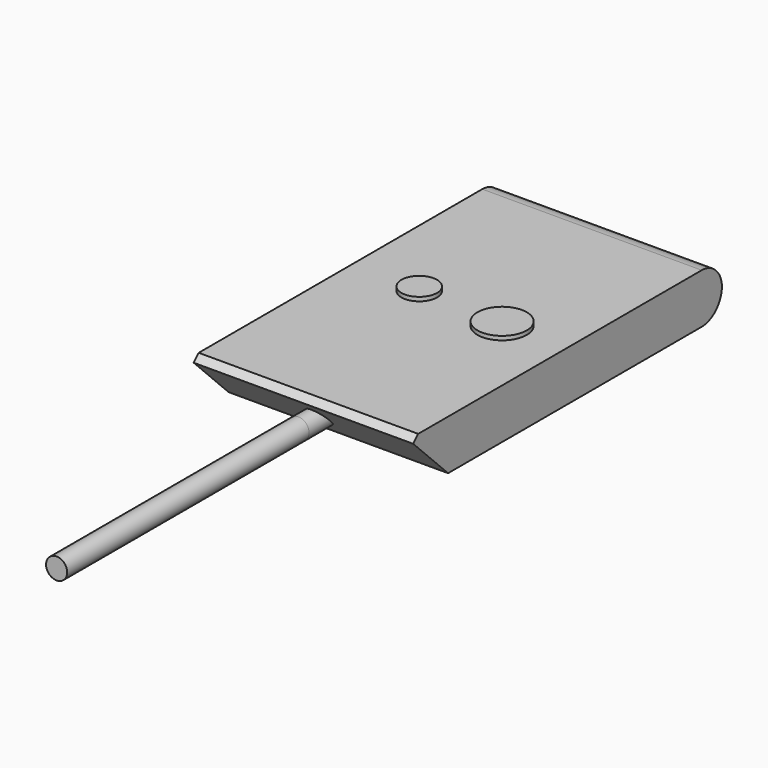
from build123d import *

# Parameters (mm, degrees)
F0_W         = 22.3715566099
F0_H         = 39.9701632559
F1_DEPTH     = 5.08
F2_R         = 5.7912
F3_DEPTH     = 0.762
F4_R         = 1.0769741324
F5_DEPTH     = 50.8
F6_R         = 1.8127400762
F6_R_2       = 2.5138312633
F7_DEPTH     = 0.4064
F8_SIZE      = 1.27
F9_T4_DEPTH  = 48.4998557676
F9_S5_R      = 1.0769741324
F9_T6_DEPTH  = 26
F10_SIZE     = 1.524
F11_T1_DEPTH = 27.632068852


# Not quite as in the source:
# - a fillet or chamfer that OpenCascade refuses, or shapes differently, is made with other operations: its cross-section is extruded or revolved along the edge and cut away or added


with BuildPart() as f1:
    # F0 (on Top) → F1 (new body)
    with BuildSketch(Plane.XY):
        Rectangle(F0_W, F0_H)
    extrude(amount=F1_DEPTH)

    # F2 (on Top) → F3 (cut)
    with BuildSketch(Plane.XY):
        Circle(F2_R)
    extrude(amount=F3_DEPTH, mode=Mode.SUBTRACT)

    # F4 (on Front) → F5 (join)
    with BuildSketch(Plane.XZ):
        with Locations((0, 2.4075380061)):
            Circle(F4_R)
    extrude(amount=F5_DEPTH)

    # F6 (on face) → F7 (join)
    with BuildSketch(Plane.XY.offset(5.08)):
        with Locations((-4.1463463567, 0.584599562)):
            Circle(F6_R)
        with Locations((4.7694612294, 0)):
            Circle(F6_R_2)
    extrude(amount=F7_DEPTH)

    # F8
    f8_edges = [f1.edges().sort_by_distance(p)[0] for p in [
        (0, -19.985082, 5.08),
    ]]
    chamfer(f8_edges, length=F8_SIZE)

    # F9: chamfer of 5.08 on 1 edges, made by hand


with BuildPart() as f9_tool2:
    # F9_s3 → F9_t4 (new body)
    with BuildSketch(Plane.YZ.offset(-24.2499278838)):
        Polygon((-19.985081628, 5.08), (-14.905081628, 0), (-19.985081628, 0), align=None)
    extrude(amount=F9_T4_DEPTH)

    # F9_s5 → F9_t6 (cut, symmetric)
    with BuildSketch(Plane.XZ.offset(17.4)):
        with Locations((0, 2.4075380061)):
            Circle(F9_S5_R)
    extrude(amount=F9_T6_DEPTH, both=True, mode=Mode.SUBTRACT)


with BuildPart() as f1_1:
    add(f1.part)

    # F9_t1: cut F9_tool2
    add(f9_tool2.part, mode=Mode.SUBTRACT)

    # F10
    f10_edges = [f1_1.edges().sort_by_distance(p)[0] for p in [
        (0, 19.985082, 5.08),
        (0, 19.985082, 0),
    ]]
    chamfer(f10_edges, length=F10_SIZE)

    # F11: fillet of radius 2.54 on 4 edges, made by hand

    # F11_s2 → F11_t1 (cut)
    with BuildSketch(Plane.YZ.offset(-13.816034426)):
        with BuildLine():
            ThreePointArc((17.4089791795, 5.08), (18.3809950977, 4.8866540126), (19.2050304038, 4.3360512242))
            Line((19.2050304038, 4.3360512242), (18.461081628, 5.08))
            Line((18.461081628, 5.08), (17.4089791795, 5.08))
        make_face()
        with BuildLine():
            ThreePointArc((19.2411328522, 4.2999487758), (19.7917356405, 3.4759134698), (19.985081628, 2.5038975516))
            Line((19.985081628, 2.5038975516), (19.985081628, 3.556))
            Line((19.985081628, 3.556), (19.2411328522, 4.2999487758))
        make_face()
        with BuildLine():
            ThreePointArc((19.2411328522, 0.7800512242), (19.7917356405, 1.6040865302), (19.985081628, 2.5761024484))
            Line((19.985081628, 2.5761024484), (19.985081628, 1.524))
            Line((19.985081628, 1.524), (19.2411328522, 0.7800512242))
        make_face()
        with BuildLine():
            ThreePointArc((17.4089791795, 0), (18.3809950977, 0.1933459874), (19.2050304038, 0.7439487758))
            Line((19.2050304038, 0.7439487758), (18.461081628, 0))
            Line((18.461081628, 0), (17.4089791795, 0))
        make_face()
    extrude(amount=F11_T1_DEPTH, mode=Mode.SUBTRACT)


solid = f1_1.part
